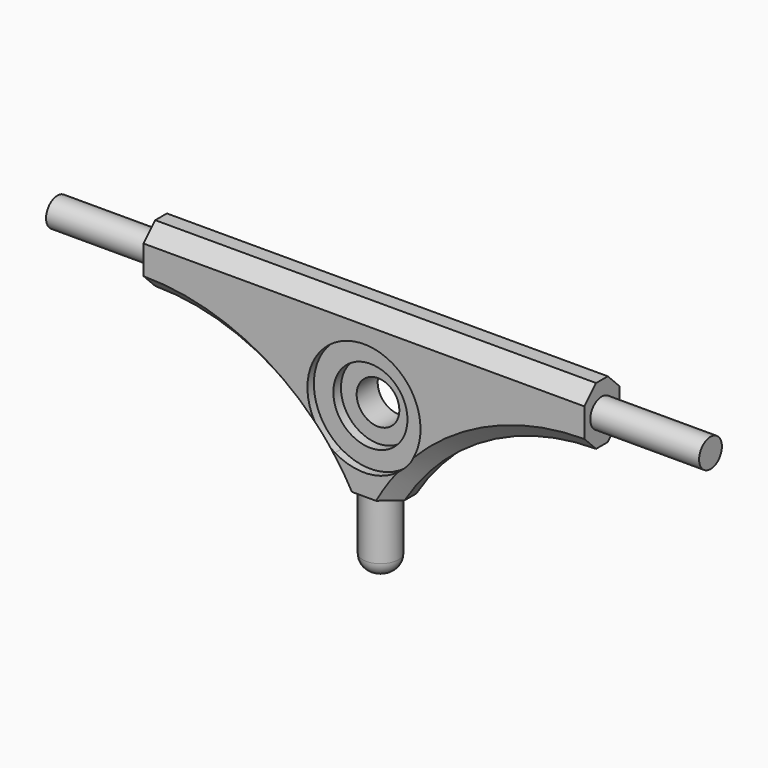
from build123d import *

# Parameters (mm, degrees)
F1_DEPTH      = 15.24
F2_R          = 6.1961301732
F3_DEPTH      = 25.4
F4_R          = 5.08
F5_R          = 4.9576785655
F6_DEPTH      = 37.846
F6_DEPTH_BACK = 189.23
F7_R          = 20.3717092778
F8_DEPTH      = 12.446
F9_R          = 12.889258446
F10_DEPTH     = 7.874
F11_R         = 13.1511811708
F12_DEPTH     = 5.08
F14_R         = 14.9583115279
F13_R         = 7.4216902204
F15_DEPTH     = 9.144
F16_DEPTH     = 47.752
F17_T1_DEPTH  = 179.4321309735
F17_T6_ANGLE  = 77.8608670263
F17_T11_ANGLE = 77.8608670263
F17_T16_ANGLE = 77.8608670263
F17_T21_ANGLE = 77.8608670263


# Not quite as in the source:
# - a fillet or chamfer that OpenCascade refuses, or shapes differently, is made with other operations: its cross-section is extruded or revolved along the edge and cut away or added


with BuildPart() as f1:
    # F0 (on Front) → F1 (new body)
    with BuildSketch(Plane.XZ):
        with BuildLine():
            Line((-76.6519159079, 10.0742522627), (-76.6519159079, -10.0742522627))
            Line((-76.6519159079, -10.0742522627), (-16.654799417, -10.0742522627))
            ThreePointArc((-16.654799417, -10.0742522627), (-13.7464055669, -6.4661247251), (-10.0742522627, -3.6390008817))
            Line((-10.0742522627, -3.6390008817), (-10.0742522627, 10.0742522627))
            Line((-10.0742522627, 10.0742522627), (-76.6519159079, 10.0742522627))
        make_face()
        with BuildLine():
            Line((-16.654799417, -10.0742522627), (-76.6519159079, -10.0742522627))
            ThreePointArc((-76.6519159079, -10.0742522627), (-38.4695929071, -20.0651922972), (-10.0742522627, -47.4771112778))
            Line((-10.0742522627, -47.4771112778), (-10.0742522627, -37.4067952444))
            ThreePointArc((-10.0742522627, -37.4067952444), (-19.1148509643, -25.124964479), (-16.654799417, -10.0742522627))
        make_face()
        with BuildLine():
            Line((10.0742522627, 10.0742522627), (10.0742522627, -3.6390008817))
            ThreePointArc((10.0742522627, -3.6390008817), (13.7464055669, -6.4661247251), (16.654799417, -10.0742522627))
            Line((16.654799417, -10.0742522627), (76.6519159079, -10.0742522627))
            Line((76.6519159079, -10.0742522627), (76.6519159079, 10.0742522627))
            Line((76.6519159079, 10.0742522627), (10.0742522627, 10.0742522627))
        make_face()
        with BuildLine():
            Line((10.0742522627, -37.4067952444), (10.0742522627, -47.4771112778))
            ThreePointArc((10.0742522627, -47.4771112778), (38.4695929071, -20.0651922972), (76.6519159079, -10.0742522627))
            Line((76.6519159079, -10.0742522627), (16.654799417, -10.0742522627))
            ThreePointArc((16.654799417, -10.0742522627), (18.8945394345, -15.0866381133), (19.6610412411, -20.5228980631))
            ThreePointArc((19.6610412411, -20.5228980631), (17.0971756716, -30.230787985), (10.0742522627, -37.4067952444))
        make_face()
        with BuildLine():
            Line((-10.0742522627, 10.0742522627), (-10.0742522627, -3.6390008817))
            ThreePointArc((-10.0742522627, -3.6390008817), (0, -0.861856822), (10.0742522627, -3.6390008817))
            Line((10.0742522627, -3.6390008817), (10.0742522627, 10.0742522627))
            Line((10.0742522627, 10.0742522627), (-10.0742522627, 10.0742522627))
        make_face()
        with BuildLine():
            Line((-10.0742522627, -37.4067952444), (-10.0742522627, -47.4771112778))
            Line((-10.0742522627, -47.4771112778), (10.0742522627, -47.4771112778))
            Line((10.0742522627, -47.4771112778), (10.0742522627, -37.4067952444))
            ThreePointArc((10.0742522627, -37.4067952444), (0, -40.1839393041), (-10.0742522627, -37.4067952444))
        make_face()
    extrude(amount=F1_DEPTH)

    # F2 (on face) → F3 (join)
    with BuildSketch(Plane(origin=(0, 0, -47.4771112778), x_dir=(1, 0, 0), z_dir=(0, 0, -1))):
        with Locations((0, 8.0302003771)):
            Circle(F2_R)
    extrude(amount=F3_DEPTH)

    # F4
    f4_edges = [f1.edges().sort_by_distance(p)[0] for p in [
        (-6.19613, -8.0302, -72.877111),
    ]]
    fillet(f4_edges, radius=F4_R)

    # F17: chamfer of 5.08 on 6 edges, made by hand

    # F17_s2 → F17_t1 (cut)
    with BuildSketch(Plane.YZ.offset(-89.7160654867)):
        Polygon((-15.24, 4.9942522627), (-10.16, 10.0742522627), (-15.24, 10.0742522627), align=None)
        Polygon((0, 4.9942522627), (-5.08, 10.0742522627), (0, 10.0742522627), align=None)
    extrude(amount=F17_T1_DEPTH, mode=Mode.SUBTRACT)


with BuildPart() as f6:
    # F5 (on face) → F6 (new body, two sides)
    with BuildSketch(Plane.YZ.offset(76.6519159079)) as f6_sk:
        with Locations((-7.7381939627, 0)):
            Circle(F5_R)
    extrude(amount=F6_DEPTH)
    extrude(f6_sk.sketch, amount=-F6_DEPTH_BACK)

    # F7 (on Front) → F8 (join)
    with BuildSketch(Plane.XZ):
        with Locations((0, -20.9111645818)):
            Circle(F7_R)
    extrude(amount=F8_DEPTH)

    # F9 (on face) → F10 (cut)
    with BuildSketch(Plane.XZ.offset(12.446)):
        with Locations((0, -20.9111645818)):
            Circle(F9_R)
    extrude(amount=-F10_DEPTH, mode=Mode.SUBTRACT)

    # F11 (on face) → F12 (cut)
    with BuildSketch(Plane(origin=(0, 0, 0), x_dir=(-1, 0, 0), z_dir=(0, 1, 0))):
        with Locations((0, -20.9111645818)):
            Circle(F11_R)
    extrude(amount=-F12_DEPTH, mode=Mode.SUBTRACT)

    # F14 (on face) + F13 (on Front) → F15 (join)
    with BuildSketch(Plane.XZ):
        with Locations((0, -20.5865148455)):
            Circle(F14_R)
    with BuildSketch(Plane.XZ):
        with Locations((0, -21.1705304682)):
            Circle(F13_R)
    extrude(amount=F15_DEPTH)

    # F13 (on Front) → F16 (cut)
    with BuildSketch(Plane.XZ):
        with Locations((0, -21.1705304682)):
            Circle(F13_R)
    extrude(amount=F16_DEPTH, mode=Mode.SUBTRACT)


with BuildPart() as f17_tool4:
    # F17_s5 → F17_t6 (revolve)
    with BuildSketch(Plane(origin=(-88.9987069649, 0, -15.0585411126), x_dir=(0, 1, 0), z_dir=(-0.9859859493, 0, -0.1668283783))):
        Polygon((-10.16, -3.9471238438), (-15.24, -9.0271238438), (-15.24, -3.9471238438), align=None)
    revolve(axis=Axis((-76.6519159079, -15.24, -88.0303138114), (0, 1, 0)), revolution_arc=F17_T6_ANGLE)

    split(bisect_by=Plane.XY.offset(-47.4771112778), keep=Keep.TOP)


with BuildPart() as f1_1:
    add(f1.part)

    # F17_t3: cut F17_tool4
    add(f17_tool4.part, mode=Mode.SUBTRACT)


with BuildPart() as f17_tool9:
    # F17_s10 → F17_t11 (revolve)
    with BuildSketch(Plane(origin=(-19.7713095684, 0, -49.575786093), x_dir=(0, 1, 0), z_dir=(-0.3704374447, 0, -0.9288574162))):
        Polygon((-15.24, 20.7723635106), (-10.16, 25.8523635106), (-15.24, 25.8523635106), align=None)
    revolve(axis=Axis((76.6519159079, -15.24, -88.0303138114), (0, 1, 0)), revolution_arc=F17_T11_ANGLE)

    split(bisect_by=Plane.XY.offset(-47.4771112778), keep=Keep.TOP)


with BuildPart() as f1_2:
    add(f1_1.part)

    # F17_t8: cut F17_tool9
    add(f17_tool9.part, mode=Mode.SUBTRACT)


with BuildPart() as f17_tool14:
    # F17_s15 → F17_t16 (revolve)
    with BuildSketch(Plane(origin=(-19.7713095684, 0, -49.575786093), x_dir=(0, 1, 0), z_dir=(-0.3704374447, 0, -0.9288574162))):
        Polygon((0, 20.7723635106), (-5.08, 25.8523635106), (0, 25.8523635106), align=None)
    revolve(axis=Axis((76.6519159079, 0, -88.0303138114), (0, 1, 0)), revolution_arc=F17_T16_ANGLE)

    split(bisect_by=Plane.XY.offset(-47.4771112778), keep=Keep.TOP)


with BuildPart() as f1_3:
    add(f1_2.part)

    # F17_t13: cut F17_tool14
    add(f17_tool14.part, mode=Mode.SUBTRACT)


with BuildPart() as f17_tool19:
    # F17_s20 → F17_t21 (revolve)
    with BuildSketch(Plane(origin=(-88.9987069649, 0, -15.0585411126), x_dir=(0, 1, 0), z_dir=(-0.9859859493, 0, -0.1668283783))):
        Polygon((-5.08, -3.9471238438), (0, -9.0271238438), (0, -3.9471238438), align=None)
    revolve(axis=Axis((-76.6519159079, 0, -88.0303138114), (0, 1, 0)), revolution_arc=F17_T21_ANGLE)

    split(bisect_by=Plane.XY.offset(-47.4771112778), keep=Keep.TOP)


with BuildPart() as f1_4:
    add(f1_3.part)

    # F17_t18: cut F17_tool19
    add(f17_tool19.part, mode=Mode.SUBTRACT)


solid = Compound([f6.part, f1_4.part])
